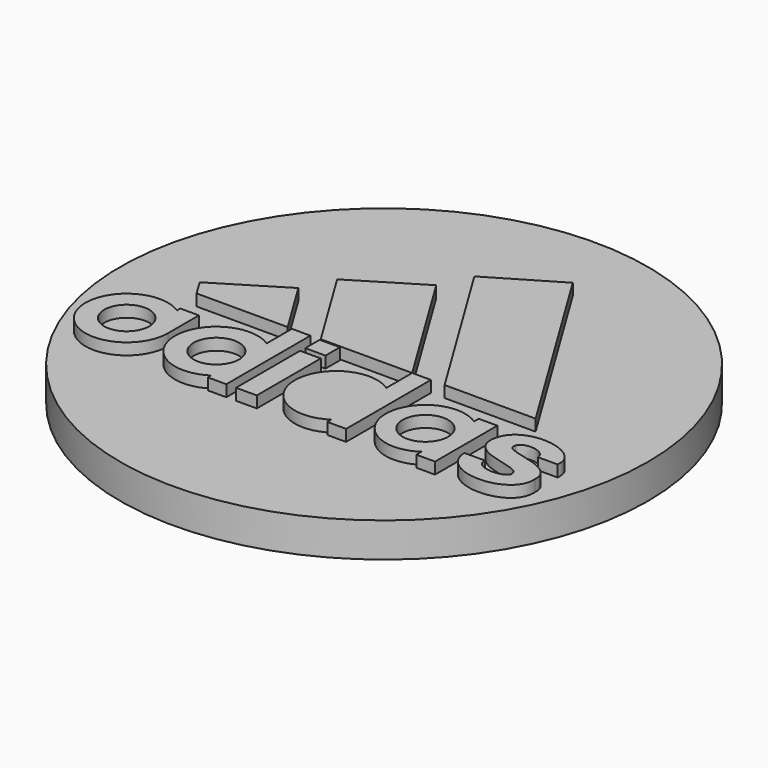
from build123d import *

# Parameters (mm, degrees)
F2_DEPTH = 25.4
F0_R     = 12.4318112904
F0_W     = 11.4617682993
F0_H     = 44.2207418382
F0_W_2   = 11.1519917846
F0_H_2   = 9.9516026676
F0_R_2   = 12.5062738248
F1_R     = 145.7892752494
F3_DEPTH = 19.05


# Not quite as in the source:
# - ends of sketch curves that miss each other by under 0.0002 mm in the source are joined


with BuildPart() as f2:
    # F0 (on Top) → F2 (new body)
    with BuildSketch(Plane.XY):
        Polygon((1.4154310087, 85.0814111872), (-35.4509100322, 63.197125618), (17.9146964107, -24.0397387488), (68.1683614854, -24.0397387488), align=None)
    extrude(amount=F2_DEPTH)



with BuildPart() as f2b:
    # F0 (on Top) → F2, piece 2 (new body)
    with BuildSketch(Plane.XY):
        Polygon((-43.1544733486, 46.5115133294), (-79.9301760288, 24.0728640339), (-50.5242412893, -23.9970767281), (-0.0220923859, -23.9970767281), align=None)
    extrude(amount=F2_DEPTH)


with BuildPart() as f2c:
    # F0 (on Top) → F2, piece 3 (new body)
    with BuildSketch(Plane.XY):
        Polygon((-87.9340324937, 7.2873335886), (-124.5343486075, -15.1022614479), (-119.0583563072, -24.0538770936), (-68.7616020441, -24.0538770936), align=None)
    extrude(amount=F2_DEPTH)


with BuildPart() as f2d:
    # F0 (on Top) → F2, piece 4 (new body)
    with BuildSketch(Plane.XY):
        with BuildLine():
            ThreePointArc((-115.5487370206, -79.725733398), (-108.144442427, -71.5262307009), (-105.4665705219, -60.8078154744))
            ThreePointArc((-105.4665705219, -60.8078154744), (-108.197031354, -49.991301665), (-115.7341323928, -41.7666743011))
            ThreePointArc((-115.7341323928, -41.7666743011), (-151.045559868, -60.9191207004), (-115.5487370206, -79.725733398))
        make_face()
        with Locations((-128.2562011003, -60.8078154744)):
            Circle(F0_R, mode=Mode.SUBTRACT)
        with BuildLine():
            ThreePointArc((-115.7341323928, -41.7666743011), (-108.197031354, -49.991301665), (-105.4665705219, -60.8078154744))
            Line((-105.4665705219, -60.8078154744), (-105.4880023073, -39.4462024353))
            Line((-105.4880023073, -39.4462024353), (-115.7341323928, -39.4462024353))
            Line((-115.7341323928, -39.4462024353), (-115.7341323928, -41.7666743011))
        make_face()
    extrude(amount=F2_DEPTH)


with BuildPart() as f2e:
    # F0 (on Top) → F2, piece 5 (new body)
    with BuildSketch(Plane.XY):
        with BuildLine():
            ThreePointArc((-66.3109198213, -62.5422311202), (-91.27428841, -60.8078154744), (-66.3109198213, -59.0733998287))
            Line((-66.3109198213, -59.0733998287), (-66.3109198213, -41.6022369857))
            ThreePointArc((-66.3109198213, -41.6022369857), (-101.6047417712, -60.8078154744), (-66.3109198213, -80.0133939632))
            Line((-66.3109198213, -80.0133939632), (-66.3109198213, -62.5422311202))
        make_face()
        with BuildLine():
            Line((-66.3109198213, -24.2017358541), (-66.3109198213, -41.6022369857))
            ThreePointArc((-66.3109198213, -41.6022369857), (-59.4821948261, -48.4555819556), (-56.0976527631, -57.5189531474))
            Line((-56.0976527631, -57.5189531474), (-56.0976527631, -24.2017358541))
            Line((-56.0976527631, -24.2017358541), (-66.3109198213, -24.2017358541))
        make_face()
        with BuildLine():
            ThreePointArc((-56.0976527631, -64.0966778014), (-59.4821948261, -73.1600489933), (-66.3109198213, -80.0133939632))
            Line((-66.3109198213, -80.0133939632), (-66.3109198213, -82.260966301))
            Line((-66.3109198213, -82.260966301), (-56.0976527631, -82.260966301))
            Line((-56.0976527631, -82.260966301), (-56.0976527631, -64.0966778014))
        make_face()
        with BuildLine():
            ThreePointArc((-66.3109198213, -59.0733998287), (-66.2205777339, -59.938517056), (-66.190415346, -60.8078154744))
            ThreePointArc((-66.190415346, -60.8078154744), (-66.2205777339, -61.6771138928), (-66.3109198213, -62.5422311202))
            Line((-66.3109198213, -62.5422311202), (-66.3109198213, -80.0133939632))
            ThreePointArc((-66.3109198213, -80.0133939632), (-59.4821948261, -73.1600489933), (-56.0976527631, -64.0966778014))
            Line((-56.0976527631, -64.0966778014), (-56.0976527631, -57.5189531474))
            ThreePointArc((-56.0976527631, -57.5189531474), (-59.4821948261, -48.4555819556), (-66.3109198213, -41.6022369857))
            Line((-66.3109198213, -41.6022369857), (-66.3109198213, -59.0733998287))
        make_face()
    extrude(amount=F2_DEPTH)


with BuildPart() as f2f:
    # F0 (on Top) → F2, piece 6 (new body)
    with BuildSketch(Plane.XY):
        with Locations((-45.0087655336, -60.1198617369)):
            Rectangle(F0_W, F0_H)
    extrude(amount=F2_DEPTH)


with BuildPart() as f2g:
    # F0 (on Top) → F2, piece 7 (new body)
    with BuildSketch(Plane.XY):
        with Locations((-44.9714139104, -29.6990927309)):
            Rectangle(F0_W_2, F0_H_2)
    extrude(amount=F2_DEPTH)


with BuildPart() as f2h:
    # F0 (on Top) → F2, piece 8 (new body)
    with BuildSketch(Plane.XY):
        with BuildLine():
            Line((-0.0220923859, -79.7740438745), (-0.0220923859, -41.8415870743))
            ThreePointArc((-0.0220923859, -41.8415870743), (-35.3726807229, -60.8078154744), (-0.0220923859, -79.7740438745))
        make_face()
        with Locations((-12.6095247019, -60.8078154744)):
            Circle(F0_R_2, mode=Mode.SUBTRACT)
        with Locations((-12.6095247019, -60.8078154744)):
            Circle(F0_R_2)
        with BuildLine():
            Line((10.3136608377, -23.9970767281), (-0.0220923859, -23.9970767281))
            Line((-0.0220923859, -23.9970767281), (-0.0220923859, -41.8415870743))
            ThreePointArc((-0.0220923859, -41.8415870743), (7.4490265637, -50.0460408456), (10.1536313191, -60.8078154744))
            ThreePointArc((10.1536313191, -60.8078154744), (7.4490265637, -71.5695901032), (-0.0220923859, -79.7740438745))
            Line((-0.0220923859, -79.7740438745), (-0.0220923859, -82.5562179089))
            Line((-0.0220923859, -82.5562179089), (10.3136608377, -82.5562179089))
            Line((10.3136608377, -82.5562179089), (10.3136608377, -23.9970767281))
        make_face()
        with BuildLine():
            ThreePointArc((10.1536313191, -60.8078154744), (7.4490265637, -50.0460408456), (-0.0220923859, -41.8415870743))
            Line((-0.0220923859, -41.8415870743), (-0.0220923859, -79.7740438745))
            ThreePointArc((-0.0220923859, -79.7740438745), (7.4490265637, -71.5695901032), (10.1536313191, -60.8078154744))
        make_face()
    extrude(amount=F2_DEPTH)


with BuildPart() as f2i:
    # F0 (on Top) → F2, piece 9 (new body)
    with BuildSketch(Plane.XY):
        with BuildLine():
            ThreePointArc((49.0602143109, -58.2645321963), (49.2547882882, -59.5295636165), (49.3198706541, -60.8078154744))
            ThreePointArc((49.3198706541, -60.8078154744), (49.2547882882, -62.0860673324), (49.0602143109, -63.3510987525))
            Line((49.0602143109, -63.3510987525), (49.0602143109, -78.9162193359))
            ThreePointArc((49.0602143109, -78.9162193359), (56.0973011295, -71.05087688), (58.6397204267, -60.8078154744))
            ThreePointArc((58.6397204267, -60.8078154744), (56.0973011295, -50.5647540689), (49.0602143109, -42.699411613))
            Line((49.0602143109, -42.699411613), (49.0602143109, -58.2645321963))
        make_face()
        with BuildLine():
            ThreePointArc((49.0602143109, -63.3510987525), (24.1492502559, -60.8078154744), (49.0602143109, -58.2645321963))
            Line((49.0602143109, -58.2645321963), (49.0602143109, -42.699411613))
            ThreePointArc((49.0602143109, -42.699411613), (14.8294004833, -60.8078154744), (49.0602143109, -78.9162193359))
            Line((49.0602143109, -78.9162193359), (49.0602143109, -63.3510987525))
        make_face()
        with BuildLine():
            Line((49.0602143109, -39.4707284868), (49.0602143109, -42.699411613))
            ThreePointArc((49.0602143109, -42.699411613), (56.0973011295, -50.5647540689), (58.6397204267, -60.8078154744))
            ThreePointArc((58.6397204267, -60.8078154744), (56.0973011295, -71.05087688), (49.0602143109, -78.9162193359))
            Line((49.0602143109, -78.9162193359), (49.0602143109, -82.4721604586))
            Line((49.0602143109, -82.4721604586), (59.3724772334, -82.4721604586))
            Line((59.3724772334, -82.4721604586), (59.3724772334, -39.4707284868))
            Line((59.3724772334, -39.4707284868), (49.0602143109, -39.4707284868))
        make_face()
    extrude(amount=F2_DEPTH)


with BuildPart() as f2j:
    # F0 (on Top) → F2, piece 10 (new body)
    with BuildSketch(Plane.XY):
        with BuildLine():
            Line((75.5096077919, -68.2697445154), (64.1811043024, -68.2697445154))
            add(Edge.make_bspline(
                [(64.1811043024, -68.2697445154), (64.8614317179, -88.639266789), (104.5420496876, -88.2522910833), (103.2439946348, -68.2697445154)],
                knots=[0, 0, 0, 0, 39.0628903324, 39.0628903324, 39.0628903324, 39.0628903324], degree=3))
            add(Edge.make_bspline(
                [(103.2439946348, -68.2697445154), (104.1533201933, -52.8722066932), (73.848571464, -56.6036510117), (77.092024813, -49.228692017)],
                knots=[0, 0, 0, 0, 32.3494544902, 32.3494544902, 32.3494544902, 32.3494544902], degree=3))
            add(Edge.make_bspline(
                [(77.092024813, -49.228692017), (77.6151120663, -44.361487031), (90.9695401788, -44.7315291703), (91.360060347, -51.5239039633)],
                knots=[0, 0, 0, 0, 14.4514648351, 14.4514648351, 14.4514648351, 14.4514648351], degree=3))
            Line((91.360060347, -51.5239039633), (102.2011523787, -51.5239039633))
            add(Edge.make_bspline(
                [(102.2011523787, -51.5239039633), (105.0276011229, -35.6890372932), (66.8714791536, -29.8843532801), (65.5021527284, -51.5239039633)],
                knots=[0, 0, 0, 0, 36.6989996503, 36.6989996503, 36.6989996503, 36.6989996503], degree=3))
            add(Edge.make_bspline(
                [(65.5021527284, -51.5239039633), (65.4783546925, -65.2542263269), (86.2978249788, -63.628911972), (91.3877934217, -68.2697445154)],
                knots=[0, 0, 0, 0, 30.8300108644, 30.8300108644, 30.8300108644, 30.8300108644], degree=3))
            add(Edge.make_bspline(
                [(75.5096077919, -68.2697445154), (75.0243961811, -77.4975006037), (97.3227471113, -75.3631476813), (91.3877934217, -68.2697445154)],
                knots=[0, 0, 0, 0, 15.8781856298, 15.8781856298, 15.8781856298, 15.8781856298], degree=3))
        make_face()
    extrude(amount=F2_DEPTH)


with BuildPart() as f2_1:
    add(f2.part)

    add(f2c.part)  # F3 merges F2c

    add(f2d.part)  # F3 merges F2d

    add(f2e.part)  # F3 merges F2e

    add(f2f.part)  # F3 merges F2f

    add(f2g.part)  # F3 merges F2g

    add(f2h.part)  # F3 merges F2h

    add(f2i.part)  # F3 merges F2i

    add(f2j.part)  # F3 merges F2j
    # F1 (on Top) → F3 (join)
    with BuildSketch(Plane.XY):
        with Locations((-22.1383590251, -15.7661773264)):
            Circle(F1_R)
    extrude(amount=F3_DEPTH)


solid = Compound([f2b.part, f2_1.part])
